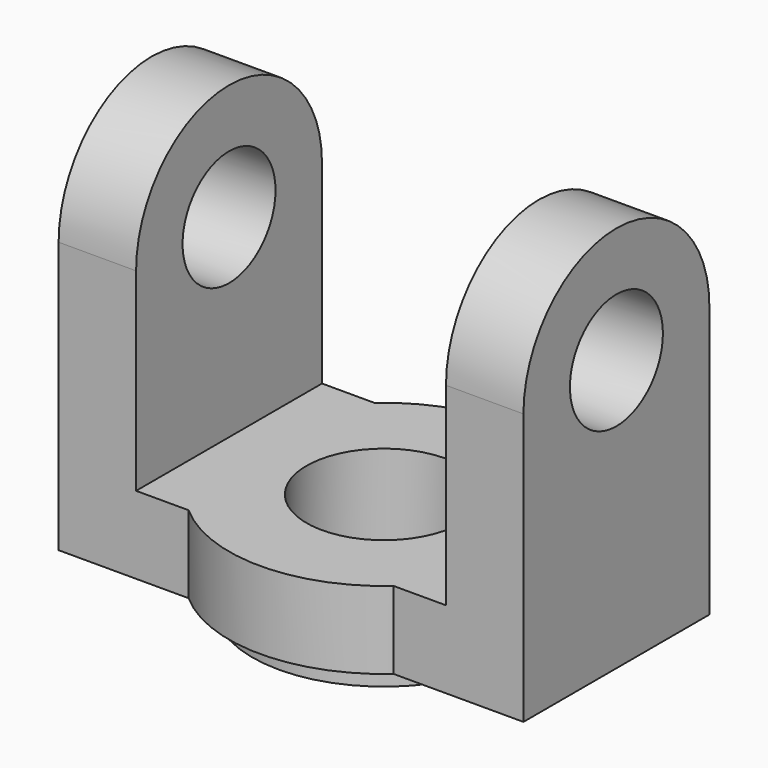
from build123d import *

# Parameters (mm, degrees)
F0_R     = 10
F1_DEPTH = 10
F2_W     = 10
F2_H     = 30
F3_DEPTH = 50
F4_R     = 7.5
F5_DEPTH = 60.001
F6_R     = 17
F6_R_2   = 10
F7_DEPTH = 3


with BuildPart() as f1:
    # F0 (on Top) → F1 (new body)
    with BuildSketch(Plane.XY):
        with BuildLine():
            Line((13.2287565553, 15), (0, 15))
            Line((0, 15), (-13.2287565553, 15))
            ThreePointArc((-13.2287565553, 15), (-20, 0), (-13.2287565553, -15))
            Line((-13.2287565553, -15), (0, -15))
            Line((0, -15), (13.2287565553, -15))
            ThreePointArc((13.2287565553, -15), (18.2287565553, -8.2287565553), (20, 0))
            ThreePointArc((20, 0), (18.2287565553, 8.2287565553), (13.2287565553, 15))
        make_face()
        Circle(F0_R, mode=Mode.SUBTRACT)
        with BuildLine():
            Line((30, 15), (13.2287565553, 15))
            ThreePointArc((13.2287565553, 15), (18.2287565553, 8.2287565553), (20, 0))
            ThreePointArc((20, 0), (18.2287565553, -8.2287565553), (13.2287565553, -15))
            Line((13.2287565553, -15), (30, -15))
            Line((30, -15), (30, 15))
        make_face()
        with BuildLine():
            ThreePointArc((-13.2287565553, -15), (-20, 0), (-13.2287565553, 15))
            Line((-13.2287565553, 15), (-30, 15))
            Line((-30, 15), (-30, -15))
            Line((-30, -15), (-13.2287565553, -15))
        make_face()
        with BuildLine():
            Line((-13.2287565553, 15), (0, 15))
            Line((0, 15), (13.2287565553, 15))
            ThreePointArc((13.2287565553, 15), (0, 20), (-13.2287565553, 15))
        make_face()
        with BuildLine():
            Line((0, -15), (-13.2287565553, -15))
            ThreePointArc((-13.2287565553, -15), (0, -20), (13.2287565553, -15))
            Line((13.2287565553, -15), (0, -15))
        make_face()
    extrude(amount=F1_DEPTH)

    # F2 (on face) → F3 (join)
    with BuildSketch(Plane.XY.offset(10)):
        with Locations((25, 0)):
            Rectangle(F2_W, F2_H)
        with Locations((-25, 0)):
            Rectangle(F2_W, F2_H)
    extrude(amount=F3_DEPTH)

    # F4 (on face) → F5 (cut, through all)
    with BuildSketch(Plane.YZ.offset(30)):
        with BuildLine():
            Line((-15, 60), (-15, 35))
            ThreePointArc((-15, 35), (0, 50), (15, 35))
            Line((15, 35), (15, 60))
            Line((15, 60), (-15, 60))
        make_face()
        with Locations((0, 35)):
            Circle(F4_R)
    extrude(amount=-F5_DEPTH, mode=Mode.SUBTRACT)

    # F6 (on face) → F7 (join)
    with BuildSketch(Plane(origin=(0, 0, 0), x_dir=(1, 0, 0), z_dir=(0, 0, -1))):
        Circle(F6_R)
        Circle(F6_R_2, mode=Mode.SUBTRACT)
    extrude(amount=F7_DEPTH)


solid = f1.part
